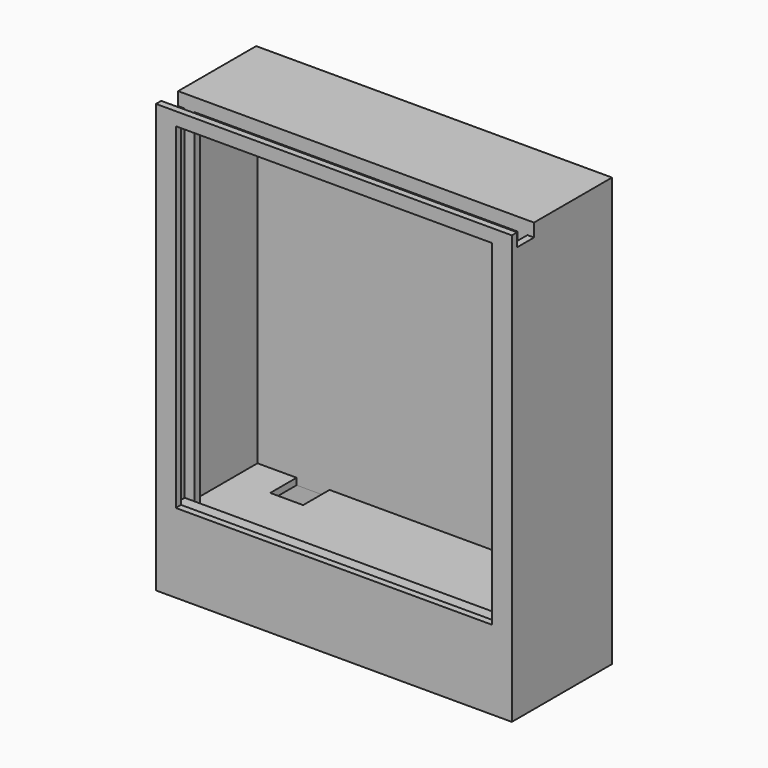
from build123d import *

# Parameters (mm, degrees)
F0_W      = 54
F0_H      = 19
F1_DEPTH  = 10
F2_W      = 1
F2_H      = 51
F3_DEPTH  = 3
F2_H_2    = 1
F4_DEPTH  = 1
F2_H_3    = 54
F5_DEPTH  = 54
F2_W_2    = 3.2
F6_DEPTH  = 1
F2_H_4    = 2
F7_DEPTH  = 54
F8_DEPTH  = 2.5
F10_W     = 2
F10_H     = 2.8
F11_DEPTH = 18
F12_W     = 2
F12_H     = 2.8
F13_DEPTH = 4.5
F14_DEPTH = 1
F15_DEPTH = 5
F16_W     = 5
F16_H     = 5
F17_DEPTH = 1


# Not quite as in the source:
# - a feature names something its author has since deleted; it is built from what else it names


with BuildPart() as f1:
    # F0 (on Top) → F1 (new body)
    with BuildSketch(Plane.XY):
        Rectangle(F0_W, F0_H)
    extrude(amount=F1_DEPTH)

    # F2 (on face) → F3 (join)
    with BuildSketch(Plane.YZ.offset(27)):
        with Locations((-9, 37.5)):
            Rectangle(F2_W, F2_H)
        Polygon((-9.5, 12), (-9.5, 10), (-8.5, 10), (-8.5, 11), (-8.5, 12), align=None)
    extrude(amount=-F3_DEPTH)

    # F2 (on face) → F4 (join)
    with BuildSketch(Plane.YZ.offset(27)):
        Polygon((-5.3, 11), (-5.3, 10), (-4.3, 10), (-4.3, 63), (-5.3, 63), align=None)
        Polygon((-4.3, 63), (-4.3, 10), (8.5, 10), (8.5, 64), (-4.3, 64), align=None)
        with Locations((-4.8, 63.5)):
            Rectangle(F2_W, F2_H_2)
    extrude(amount=-F4_DEPTH)

    # F2 (on face) → F5 (join, through all)
    with BuildSketch(Plane.YZ.offset(27)):
        with Locations((9, 37)):
            Rectangle(F2_W, F2_H_3)
        Polygon((8.5, 64), (9.5, 64), (9.5, 65), (-5.3, 65), (-5.3, 64), (-4.3, 64), align=None)
    extrude(amount=-F5_DEPTH)

    # F2 (on face) → F6 (join)
    with BuildSketch(Plane.YZ.offset(27)):
        Polygon((-8.5, 12), (-8.5, 11), (-5.3, 11), (-5.3, 63), (-8.5, 63), align=None)
        with Locations((-6.9, 10.5)):
            Rectangle(F2_W_2, F2_H_2)
    extrude(amount=-F6_DEPTH)

    # F2 (on face) → F7 (join, through all)
    with BuildSketch(Plane.YZ.offset(27)):
        with Locations((-6.9, 10.5)):
            Rectangle(F2_W_2, F2_H_2)
        Polygon((-9.5, 12), (-9.5, 10), (-8.5, 10), (-8.5, 11), (-8.5, 12), align=None)
        with Locations((-4.8, 63.5)):
            Rectangle(F2_W, F2_H_2)
        with Locations((-9, 64)):
            Rectangle(F2_W, F2_H_4)
    extrude(amount=-F7_DEPTH)

    # F2 (on face) → F8 (join)
    with BuildSketch(Plane.YZ.offset(27)):
        Polygon((-5.3, 11), (-5.3, 10), (-4.3, 10), (-4.3, 63), (-5.3, 63), align=None)
    extrude(amount=-F8_DEPTH)

    # F9: F1 across plane


with BuildPart() as f1_1:
    add(f1.part)
    add(f1.part.mirror(Plane.YZ))

    # F10 (on face) → F11 (cut)
    with BuildSketch(Plane(origin=(0, 9.5, 0), x_dir=(-1, 0, 0), z_dir=(0, 1, 0))):
        with Locations((26, 6.6)):
            Rectangle(F10_W, F10_H)
        Polygon((25, 3.7), (25, 5.2), (25, 8), (25, 9), (2.5, 9), (2.5, 8), (2.5, 3.7), align=None)
    extrude(amount=-F11_DEPTH, mode=Mode.SUBTRACT)

    # F12 (on face) → F13 (join)
    with BuildSketch(Plane(origin=(0, -8.5, 0), x_dir=(-1, 0, 0), z_dir=(0, 1, 0))):
        with Locations((26, 6.6)):
            Rectangle(F12_W, F12_H)
    extrude(amount=F13_DEPTH)

    # F16 (on face) → F17 (cut, through all)
    with BuildSketch(Plane.XY.offset(10)):
        with Locations((-17.5664718822, 6)):
            Rectangle(F16_W, F16_H)
    extrude(amount=-F17_DEPTH, mode=Mode.SUBTRACT)


with BuildPart() as f14:
    # F10 (on face) → F14 (new body)
    with BuildSketch(Plane(origin=(0, 9.5, 0), x_dir=(-1, 0, 0), z_dir=(0, 1, 0))):
        Polygon((25, 3.7), (25, 5.2), (25, 8), (25, 9), (2.5, 9), (2.5, 8), (2.5, 3.7), align=None)
    extrude(amount=-F14_DEPTH)

    # F10 (on face) → F15 (join)
    with BuildSketch(Plane(origin=(0, 9.5, 0), x_dir=(-1, 0, 0), z_dir=(0, 1, 0))):
        with Locations((26, 6.6)):
            Rectangle(F10_W, F10_H)
    extrude(amount=-F15_DEPTH)


solid = Compound([f1_1.part, f14.part])
